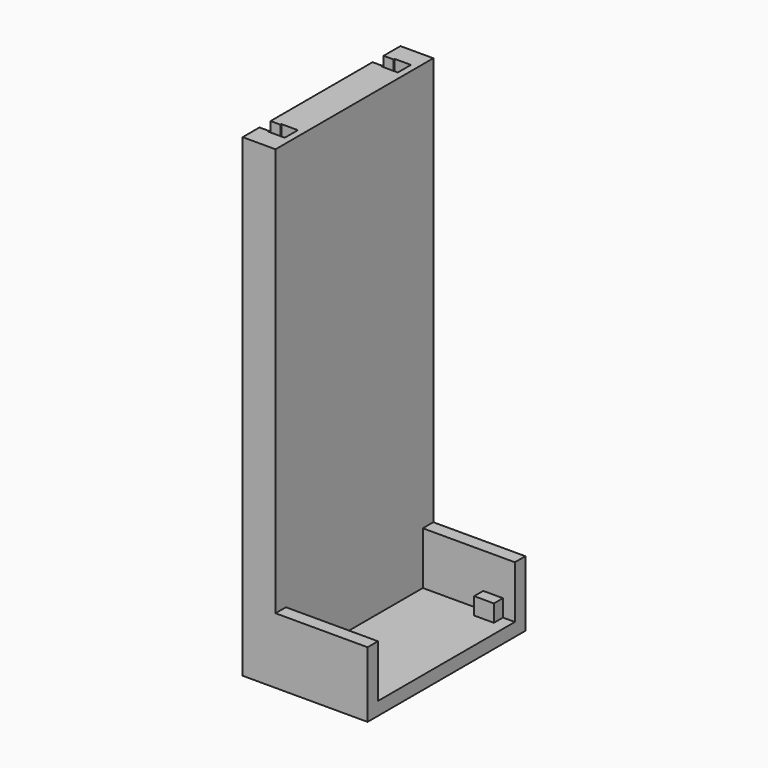
from build123d import *

# Parameters (mm, degrees)
F1_DEPTH  = 76.2
F3_DEPTH  = 25.4
F4_DEPTH  = 5.08
F5_W      = 7.62
F5_H      = 4.3815
F6_DEPTH  = 11.684
F7_W      = 6.35
F7_H      = 6.35
F8_DEPTH  = 55.88
F9_W      = 5.334
F9_H      = 5.334
F10_DEPTH = 5.08


# Not quite as in the source:
# - a feature names something its author has since deleted; it is built from what else it names


with BuildPart() as f1:
    # F0 (on Front) → F1 (new body)
    with BuildSketch(Plane.XZ):
        Polygon((0, 0), (12.7, 0), (12.7, 5.4184001555), (12.7, 23.5612627981), (12.7, 183.226400471), (0, 183.226400471), align=None)
    extrude(amount=F1_DEPTH)

    # F2 (on Top) → F3 (join)
    with BuildSketch(Plane.XY):
        Polygon((43.18, 0), (0, 0), (0, -5.0670392811), (48.26, -5.0670392811), (48.26, 0), align=None)
        Polygon((27.7881938964, -71.1809098721), (0, -71.1809098721), (0, -76.2), (30.48, -76.2), (48.26, -76.2), (48.26, -71.1809098721), (35.56, -71.1809098721), align=None)
    extrude(amount=F3_DEPTH)

    # F2 (on Top) → F4 (join)
    with BuildSketch(Plane.XY):
        Polygon((43.18, 0), (0, 0), (0, -5.0670392811), (48.26, -5.0670392811), (48.26, 0), align=None)
        Polygon((48.26, -5.0670392811), (0, -5.0670392811), (0, -71.1809098721), (27.7881938964, -71.1809098721), (35.56, -71.1809098721), (48.26, -71.1809098721), align=None)
    extrude(amount=F4_DEPTH)

    # F5 (on Top) → F6 (join)
    with BuildSketch(Plane.XY):
        with Locations((39.8590039933, -7.2577892811)):
            Rectangle(F5_W, F5_H)
        with Locations((39.8590039933, -68.9901598721)):
            Rectangle(F5_W, F5_H)
    extrude(amount=F6_DEPTH)

    # F7 (on face) → F8 (cut)
    with BuildSketch(Plane.XY.offset(183.226400471)):
        with Locations((6.985, -10.795)):
            Rectangle(F7_W, F7_H)
        with Locations((6.985, -65.405)):
            Rectangle(F7_W, F7_H)
    extrude(amount=-F8_DEPTH, mode=Mode.SUBTRACT)

    # F9 (on Right) → F10 (cut)
    with BuildSketch(Plane.YZ):
        with Locations((-65.405, 180.559400471)):
            Rectangle(F9_W, F9_H)
        with Locations((-10.795, 180.559400471)):
            Rectangle(F9_W, F9_H)
    extrude(amount=F10_DEPTH, mode=Mode.SUBTRACT)


solid = f1.part
